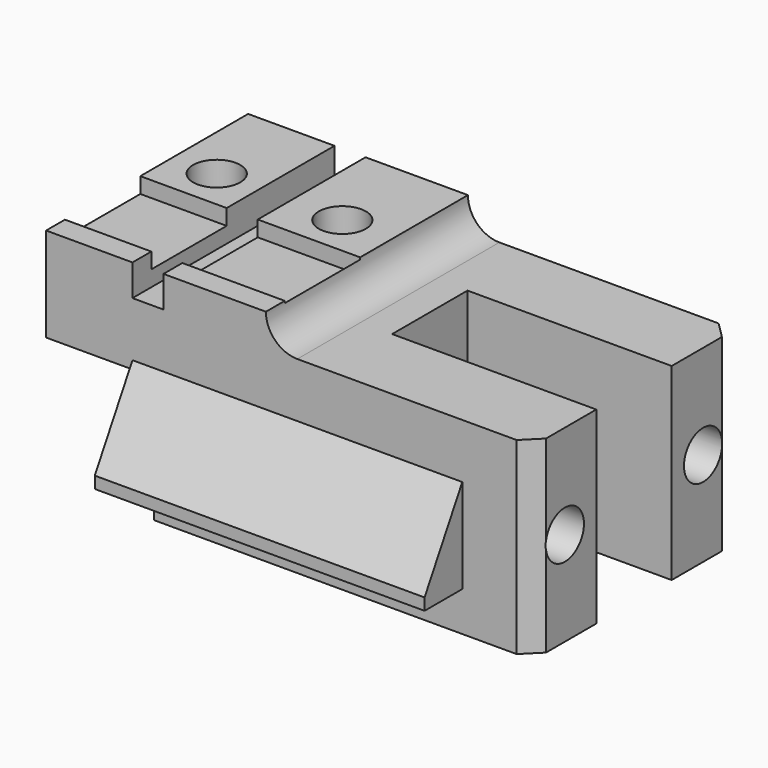
from build123d import *

# Parameters (mm, degrees)
F1_DEPTH  = 51.054
F2_R      = 6.34999
F3_W      = 41.275
F3_H      = 19.05
F4_DEPTH  = 76.2
F5_SIZE2  = 3.302
F5_SIZE   = 3.302
F6_W      = 44.45
F6_H      = 19.05
F7_DEPTH  = 3.175
F8_R      = 4.826
F9_DEPTH  = 16.002
F10_R     = 4.7625
F11_DEPTH = 12.7
F12_W     = 66.675
F12_H     = 19.05
F13_DEPTH = 9.525
F15_DEPTH = 76.2
F16_W     = 67.945
F16_H     = 19.05
F17_DEPTH = 9.525
F19_DEPTH = 85.4085


# Not quite as in the source:
# - a fillet or chamfer is up to 0.001 mm smaller than in the source, because OpenCascade refuses the exact size


with BuildPart() as f1:
    # F0 (on Front) → F1 (new body)
    with BuildSketch(Plane.XZ):
        Polygon((-38.7827743664, 8.7870896519), (-16.9203323245, 8.7870896519), (-16.9203323245, -16.6129103481), (59.6422256336, -16.6129103481), (59.6422256336, 21.4870896519), (5.6545256336, 21.4870896519), (5.6545256336, 27.8370896519), (-15.0464743664, 27.8370896519), (-15.0464743664, 21.4870896519), (-21.3202743664, 21.4870896519), (-21.3202743664, 27.8370896519), (-38.7827743664, 27.8370896519), align=None)
    extrude(amount=F1_DEPTH)

    # F2 (radius 6.35 in the source; OpenCascade refuses exactly that, so slightly less here)
    f2_edges = [f1.edges().sort_by_distance(p)[0] for p in [
        (5.654526, -25.527, 21.48709),
    ]]
    fillet(f2_edges, radius=F2_R)

    # F3 (on face) → F4 (cut)
    with BuildSketch(Plane.XY.offset(21.4870896519)):
        with Locations((39.0047256336, -25.527)):
            Rectangle(F3_W, F3_H)
    extrude(amount=-F4_DEPTH, mode=Mode.SUBTRACT)

    # F5
    f5_edges = [f1.edges().sort_by_distance(p)[0] for p in [
        (59.642226, -51.054, 2.43709),
        (59.642226, 0, 2.43709),
    ]]
    chamfer(f5_edges, length=F5_SIZE, length2=F5_SIZE2)

    # F6 (on face) → F7 (cut)
    with BuildSketch(Plane.XY.offset(27.8370896519)):
        with Locations((-16.5577743664, -36.7665)):
            Rectangle(F6_W, F6_H)
    extrude(amount=-F7_DEPTH, mode=Mode.SUBTRACT)

    # F8 (on face) → F9 (cut)
    with BuildSketch(Plane.YZ.offset(59.6422256336)):
        with Locations((-42.9895, 2.4370896519)):
            Circle(F8_R)
        with Locations((-8.0645, 2.4370896519)):
            Circle(F8_R)
    extrude(amount=-F9_DEPTH, mode=Mode.SUBTRACT)

    # F10 (on face) → F11 (cut)
    with BuildSketch(Plane.XY.offset(27.8370896519)):
        with Locations((-29.8927743664, -19.05)):
            Circle(F10_R)
        with Locations((-4.4927743664, -19.05)):
            Circle(F10_R)
    extrude(amount=-F11_DEPTH, mode=Mode.SUBTRACT)

    # F12 (on face) → F13 (join)
    with BuildSketch(Plane.XZ.offset(51.054)):
        with Locations((12.0172256336, 0.9130896519)):
            Rectangle(F12_W, F12_H)
    extrude(amount=F13_DEPTH)

    # F14 (on face) → F15 (cut)
    with BuildSketch(Plane.YZ.offset(45.3547256336)):
        Polygon((-60.579, -6.2306603481), (-51.054, 10.4380896519), (-60.579, 10.4380896519), align=None)
    extrude(amount=-F15_DEPTH, mode=Mode.SUBTRACT)

    # F16 (on face) → F17 (join)
    with BuildSketch(Plane(origin=(0, 0, 0), x_dir=(-1, 0, 0), z_dir=(0, 1, 0))):
        with Locations((-12.6522256336, 0.9130896519)):
            Rectangle(F16_W, F16_H)
    extrude(amount=F17_DEPTH)

    # F18 (on face) → F19 (cut, through all)
    with BuildSketch(Plane.YZ.offset(46.6247256336)):
        Polygon((0, 10.4380896519), (9.525, -6.2306603481), (9.525, 10.4380896519), align=None)
    extrude(amount=-F19_DEPTH, mode=Mode.SUBTRACT)


solid = f1.part
